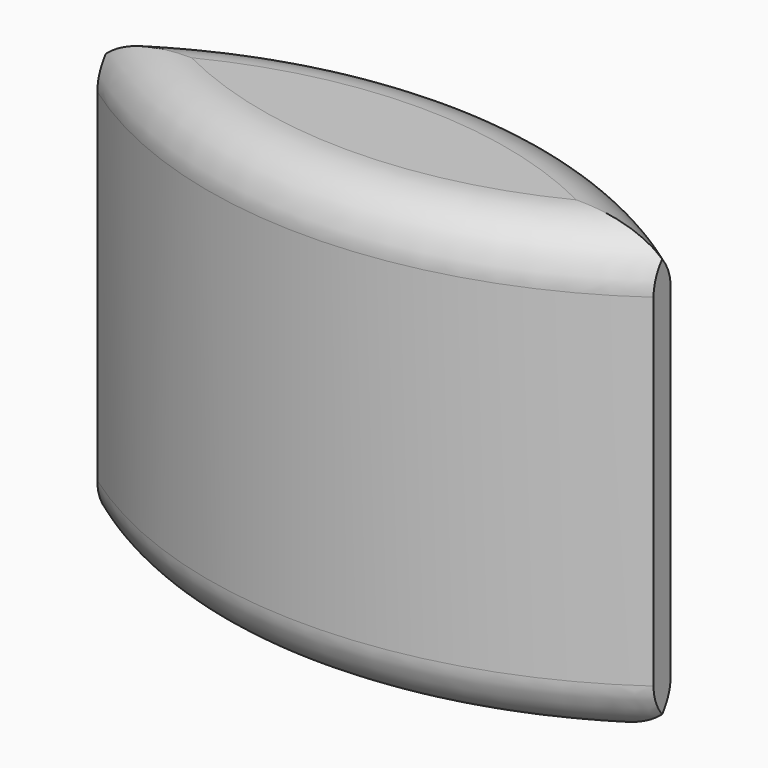
from build123d import *

# Parameters (mm, degrees)
F0_W        = 520
F0_H        = 20
F1_DEPTH    = 420
F2_T2_ANGLE = 102.4276429989
F2_T4_ANGLE = 102.4276429989
F2_T6_ANGLE = 102.4276429989
F2_T8_ANGLE = 102.4276429989


# Not quite as in the source:
# - a fillet or chamfer that OpenCascade refuses, or shapes differently, is made with other operations: its cross-section is extruded or revolved along the edge and cut away or added


with BuildPart() as f1:
    # F0 (on Top) → F1 (new body)
    with BuildSketch(Plane.XY):
        with BuildLine():
            ThreePointArc((-260, -10), (0, -92.7126465559), (260, -10))
            Line((260, -10), (-260, -10))
        make_face()
        Rectangle(F0_W, F0_H)
        with BuildLine():
            Line((-260, 10), (260, 10))
            ThreePointArc((260, 10), (0, 92.7126465559), (-260, 10))
        make_face()
    extrude(amount=F1_DEPTH)

    # F2: fillet of radius 50 on 4 edges, made by hand

    # F2_s1 → F2_t2 (revolve, cut)
    with BuildSketch(Plane(origin=(-174.4577986965, 217.0889587049, 0), x_dir=(0, 0, 1), z_dir=(-0.6264157929, 0.7794890983, 0))):
        with BuildLine():
            ThreePointArc((370, -226.1895591947), (405.3553390593, -211.544898254), (420, -176.1895591947))
            Line((420, -176.1895591947), (420, -226.1895591947))
            Line((420, -226.1895591947), (370, -226.1895591947))
        make_face()
    revolve(axis=Axis((0, 357.2873534441, 420), (0, 0, 1)), revolution_arc=F2_T2_ANGLE, mode=Mode.SUBTRACT)

    # F2_s3 → F2_t4 (revolve, cut)
    with BuildSketch(Plane(origin=(174.4577986965, -217.0889587049, 0), x_dir=(0, 0, 1), z_dir=(0.6264157929, -0.7794890983, 0))):
        with BuildLine():
            ThreePointArc((370, -226.1895591947), (405.3553390593, -211.544898254), (420, -176.1895591947))
            Line((420, -176.1895591947), (420, -226.1895591947))
            Line((420, -226.1895591947), (370, -226.1895591947))
        make_face()
    revolve(axis=Axis((0, -357.2873534441, 420), (0, 0, 1)), revolution_arc=F2_T4_ANGLE, mode=Mode.SUBTRACT)

    # F2_s5 → F2_t6 (revolve, cut)
    with BuildSketch(Plane(origin=(-174.4577986965, 217.0889587049, 0), x_dir=(0, 0, 1), z_dir=(-0.6264157929, 0.7794890983, 0))):
        with BuildLine():
            ThreePointArc((50, -226.1895591947), (14.6446609407, -211.544898254), (0, -176.1895591947))
            Line((0, -176.1895591947), (0, -226.1895591947))
            Line((0, -226.1895591947), (50, -226.1895591947))
        make_face()
    revolve(axis=Axis((0, 357.2873534441, 0), (0, 0, 1)), revolution_arc=F2_T6_ANGLE, mode=Mode.SUBTRACT)

    # F2_s7 → F2_t8 (revolve, cut)
    with BuildSketch(Plane(origin=(174.4577986965, -217.0889587049, 0), x_dir=(0, 0, 1), z_dir=(0.6264157929, -0.7794890983, 0))):
        with BuildLine():
            ThreePointArc((50, -226.1895591947), (14.6446609407, -211.544898254), (0, -176.1895591947))
            Line((0, -176.1895591947), (0, -226.1895591947))
            Line((0, -226.1895591947), (50, -226.1895591947))
        make_face()
    revolve(axis=Axis((0, -357.2873534441, 0), (0, 0, 1)), revolution_arc=F2_T8_ANGLE, mode=Mode.SUBTRACT)


solid = f1.part
